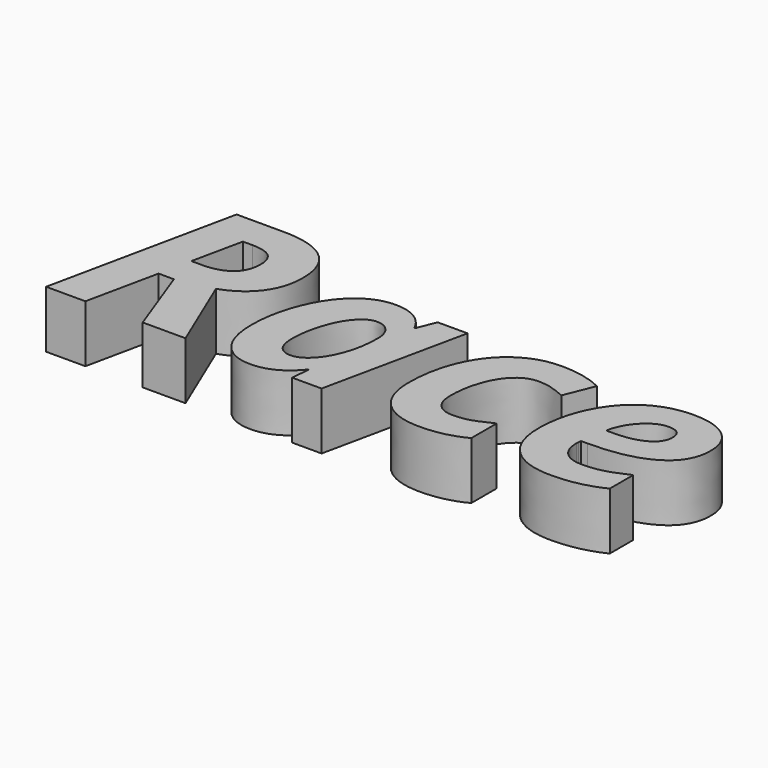
from build123d import *

# Parameters (mm, degrees)
F0_TEXT_SIZE = 117.1815829972
F1_DEPTH     = 25.4


# Not quite as in the source:
# - Text() gives the source's letters only with a copy of the font that has no kerning and outlines rounded to 1/6400 em; it was checked with that copy


with BuildPart() as f1:
    # F0 (on Top) → F1 (new body)
    with BuildSketch(Plane.XY):
        with Locations((-123.9965390414, -34.8858833313)):
            Text('Race', F0_TEXT_SIZE, font='Open Sans', font_style=FontStyle.BOLDITALIC, text_align=(TextAlign.LEFT, TextAlign.BOTTOM))
    extrude(amount=F1_DEPTH)


solid = f1.part
